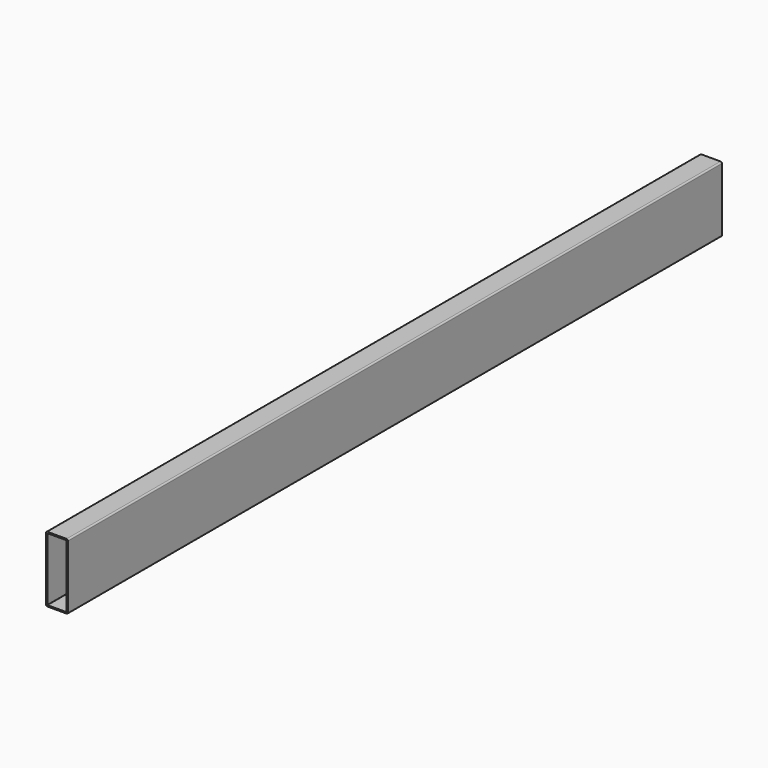
from build123d import *

# Parameters (mm, degrees)
F1_DEPTH = 946.15


# Not quite as in the source:
# - a feature names something its author has since deleted; it is built from what else it names


with BuildPart() as f1:
    # F0 (on Front) → F1 (new body)
    with BuildSketch(Plane.XZ):
        with BuildLine():
            ThreePointArc((0, 1.651), (0.4835667043, 0.4835667043), (1.651, 0))
            Line((1.651, 0), (23.749, 0))
            ThreePointArc((23.749, 0), (24.9164332957, 0.4835667043), (25.4, 1.651))
            Line((25.4, 1.651), (25.4, 74.549))
            ThreePointArc((25.4, 74.549), (24.9164332957, 75.7164332957), (23.749, 76.2))
            Line((23.749, 76.2), (1.651, 76.2))
            ThreePointArc((1.651, 76.2), (0.4835667043, 75.7164332957), (0, 74.549))
            Line((0, 74.549), (0, 1.651))
        make_face()
        with BuildLine():
            ThreePointArc((1.5240004182, 74.549), (1.5611977345, 74.6388022655), (1.651, 74.6759995818))
            Line((1.651, 74.6759995818), (23.749, 74.6759995818))
            ThreePointArc((23.749, 74.6759995818), (23.8388022655, 74.6388022655), (23.8759995818, 74.549))
            Line((23.8759995818, 74.549), (23.8759995818, 1.651))
            ThreePointArc((23.8759995818, 1.651), (23.8388022655, 1.5611977345), (23.749, 1.5240004182))
            Line((23.749, 1.5240004182), (1.651, 1.5240004182))
            ThreePointArc((1.651, 1.5240004182), (1.5611977345, 1.5611977345), (1.5240004182, 1.651))
            Line((1.5240004182, 1.651), (1.5240004182, 74.549))
        make_face(mode=Mode.SUBTRACT)
    extrude(amount=F1_DEPTH)


solid = f1.part
